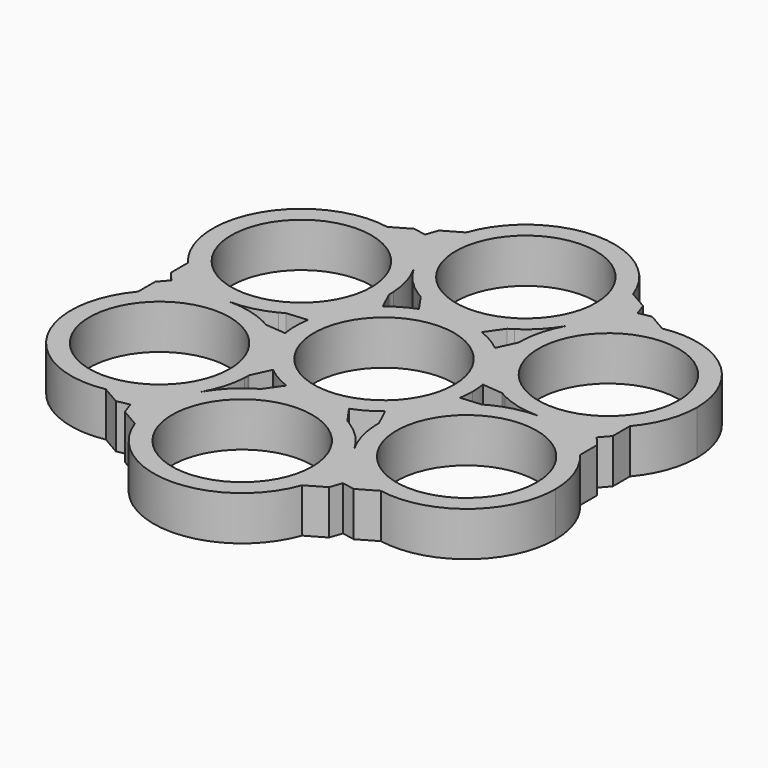
from build123d import *

# Parameters (mm, degrees)
F0_R     = 11.049
F1_DEPTH = 6.985


# Not quite as in the source:
# - a feature names something its author has since deleted; it is built from what else it names


with BuildPart() as f1:
    # F0 (on Top) → F1 (new body)
    with BuildSketch(Plane.XY):
        with BuildLine():
            ThreePointArc((13.786655701, -2.2558866507), (13.9240884826, -1.1316624621), (13.97, 0))
            ThreePointArc((13.97, 0), (13.9240884826, 1.1316624621), (13.786655701, 2.2558866507))
            ThreePointArc((13.786655701, 2.2558866507), (13.1567408564, 4.6969213362), (12.0983748352, 6.9850000964))
            ThreePointArc((12.0983748352, 6.9850000964), (10.6460235529, 9.0456112293), (8.8469829981, 10.811650745))
            ThreePointArc((8.8469829981, 10.811650745), (6.985, 12.0983748909), (4.9396727029, 13.0675373957))
            ThreePointArc((4.9396727029, 13.0675373957), (2.5107172862, 13.7425324707), (0, 13.97))
            ThreePointArc((0, 13.97), (-2.5107172862, 13.7425324707), (-4.9396727029, 13.0675373957))
            ThreePointArc((-4.9396727029, 13.0675373957), (-6.985, 12.0983748909), (-8.8469829981, 10.811650745))
            ThreePointArc((-8.8469829981, 10.811650745), (-10.6460236342, 9.0456111335), (-12.0983749609, 6.9849998787))
            ThreePointArc((-12.0983749609, 6.9849998787), (-13.1567408986, 4.6969212179), (-13.786655701, 2.2558866507))
            ThreePointArc((-13.786655701, 2.2558866507), (-13.97, 0), (-13.786655701, -2.2558866507))
            ThreePointArc((-13.786655701, -2.2558866507), (-13.1567408656, -4.6969213103), (-12.0983748628, -6.9850000487))
            ThreePointArc((-12.0983748628, -6.9850000487), (-10.6460235707, -9.0456112083), (-8.8469829981, -10.811650745))
            ThreePointArc((-8.8469829981, -10.811650745), (-6.985, -12.0983748909), (-4.9396727029, -13.0675373957))
            ThreePointArc((-4.9396727029, -13.0675373957), (-2.5107172928, -13.7425324695), (-1.35e-08, -13.97))
            ThreePointArc((-1.35e-08, -13.97), (2.5107172795, -13.7425324719), (4.9396727029, -13.0675373957))
            ThreePointArc((4.9396727029, -13.0675373957), (6.985, -12.0983748909), (8.8469829981, -10.811650745))
            ThreePointArc((8.8469829981, -10.811650745), (10.6460235529, -9.0456112293), (12.0983748352, -6.9850000964))
            ThreePointArc((12.0983748352, -6.9850000964), (13.1567408564, -4.6969213362), (13.786655701, -2.2558866507))
        make_face()
        Circle(F0_R, mode=Mode.SUBTRACT)
        with BuildLine():
            ThreePointArc((12.0983748352, 6.9850000964), (13.1567408564, 4.6969213362), (13.786655701, 2.2558866507))
            Line((13.786655701, 2.2558866507), (17.0463049997, 1.9686650985))
            ThreePointArc((17.0463049997, 1.9686650985), (14.2508878564, 4.1597639905), (12.0983748352, 6.9850000964))
        make_face()
        with BuildLine():
            Line((17.0463049997, -1.9686650985), (13.786655701, -2.2558866507))
            ThreePointArc((13.786655701, -2.2558866507), (13.1567408564, -4.6969213362), (12.0983748352, -6.9850000964))
            ThreePointArc((12.0983748352, -6.9850000964), (14.2508878564, -4.1597639905), (17.0463049997, -1.9686650985))
        make_face()
        with BuildLine():
            ThreePointArc((8.8469829981, 10.811650745), (10.6460235529, 9.0456112293), (12.0983748352, 6.9850000964))
            ThreePointArc((12.0983748352, 6.9850000964), (10.7279051882, 10.2617490221), (10.2280664867, 13.7782006212))
            Line((10.2280664867, 13.7782006212), (8.8469829981, 10.811650745))
        make_face()
        with BuildLine():
            ThreePointArc((10.2280664867, 13.7782006212), (10.7279051882, 10.2617490221), (12.0983748352, 6.9850000964))
            ThreePointArc((12.0983748352, 6.9850000964), (14.2508878564, 4.1597639905), (17.0463049997, 1.9686650985))
            ThreePointArc((17.0463049997, 1.9686650985), (17.4348836488, 1.7455136549), (17.8304191968, 1.5349392891))
            ThreePointArc((17.8304191968, 1.5349392891), (20.9223718291, 0.3891550696), (24.1967497683, 0))
            ThreePointArc((24.1967497683, 0), (30.0531688702, 1.2868120939), (34.8306887676, 4.9101853415))
            ThreePointArc((34.8306887676, 4.9101853415), (37.3062316104, 9.1427454817), (38.1667497817, 13.97))
            ThreePointArc((38.1667497817, 13.97), (33.1362668167, 24.7052659577), (21.6676896268, 27.7091686333))
            ThreePointArc((21.6676896268, 27.7091686333), (16.1409964163, 25.3834016715), (12.0983749062, 20.9550000265))
            ThreePointArc((12.0983749062, 20.9550000265), (10.7982040971, 17.9247279977), (10.244506016, 14.67412634))
            ThreePointArc((10.244506016, 14.67412634), (10.2291009922, 14.2262953244), (10.2280664867, 13.7782006212))
        make_face()
        with Locations((24.1967497817, 13.97)):
            Circle(F0_R, mode=Mode.SUBTRACT)
        with BuildLine():
            ThreePointArc((10.2280664867, -13.7782006212), (10.7279051882, -10.2617490221), (12.0983748352, -6.9850000964))
            ThreePointArc((12.0983748352, -6.9850000964), (10.6460235529, -9.0456112293), (8.8469829981, -10.811650745))
            Line((8.8469829981, -10.811650745), (10.2280664867, -13.7782006212))
        make_face()
        with BuildLine():
            ThreePointArc((17.0463049997, -1.9686650985), (14.2508878564, -4.1597639905), (12.0983748352, -6.9850000964))
            ThreePointArc((12.0983748352, -6.9850000964), (10.7279051882, -10.2617490221), (10.2280664867, -13.7782006212))
            ThreePointArc((10.2280664867, -13.7782006212), (10.2291009922, -14.2262953244), (10.244506016, -14.67412634))
            ThreePointArc((10.244506016, -14.67412634), (10.7982040928, -17.9247279832), (12.0983748911, -20.9550000004))
            ThreePointArc((12.0983748911, -20.9550000004), (16.140996404, -25.3834016628), (21.6676896268, -27.7091686333))
            ThreePointArc((21.6676896268, -27.7091686333), (33.1362668167, -24.7052659577), (38.1667497817, -13.97))
            ThreePointArc((38.1667497817, -13.97), (37.3062316104, -9.1427454817), (34.8306887676, -4.9101853415))
            ThreePointArc((34.8306887676, -4.9101853415), (30.0531688702, -1.2868120939), (24.1967497683, 0))
            ThreePointArc((24.1967497683, 0), (20.9223718291, -0.3891550696), (17.8304191968, -1.5349392891))
            ThreePointArc((17.8304191968, -1.5349392891), (17.4348836488, -1.7455136549), (17.0463049997, -1.9686650985))
        make_face()
        with Locations((24.1967497817, -13.97)):
            Circle(F0_R, mode=Mode.SUBTRACT)
        with BuildLine():
            ThreePointArc((0, 13.97), (2.5107172862, 13.7425324707), (4.9396727029, 13.0675373957))
            Line((4.9396727029, 13.0675373957), (6.818238513, 15.7468657196))
            ThreePointArc((6.818238513, 15.7468657196), (3.5229826925, 14.4215129194), (0, 13.97))
        make_face()
        with BuildLine():
            ThreePointArc((34.8306887676, 4.9101853415), (30.0531688702, 1.2868120939), (24.1967497683, 0))
            ThreePointArc((24.1967497683, 0), (30.0531688702, -1.2868120939), (34.8306887676, -4.9101853415))
            Line((34.8306887676, -4.9101853415), (34.8306887676, -1.5349392891))
            Line((34.8306887676, -1.5349392891), (33.5076935589, 0))
            Line((33.5076935589, 0), (34.8306887676, 1.5349392891))
            Line((34.8306887676, 1.5349392891), (34.8306887676, 4.9101853415))
        make_face()
        with BuildLine():
            Line((6.818238513, -15.7468657196), (4.9396727029, -13.0675373957))
            ThreePointArc((4.9396727029, -13.0675373957), (2.5107172795, -13.7425324719), (-1.35e-08, -13.97))
            ThreePointArc((-1.35e-08, -13.97), (3.5229826859, -14.4215129177), (6.818238513, -15.7468657196))
        make_face()
        with BuildLine():
            ThreePointArc((-4.9396727029, 13.0675373957), (-2.5107172862, 13.7425324707), (0, 13.97))
            ThreePointArc((0, 13.97), (-3.5229826925, 14.4215129194), (-6.818238513, 15.7468657196))
            Line((-6.818238513, 15.7468657196), (-4.9396727029, 13.0675373957))
        make_face()
        with BuildLine():
            ThreePointArc((-6.818238513, 15.7468657196), (-3.5229826925, 14.4215129194), (0, 13.97))
            ThreePointArc((0, 13.97), (3.5229826925, 14.4215129194), (6.818238513, 15.7468657196))
            ThreePointArc((6.818238513, 15.7468657196), (7.2057826566, 15.9718089794), (7.5859131808, 16.2090656291))
            ThreePointArc((7.5859131808, 16.2090656291), (10.1241677534, 18.3138830621), (12.0983749062, 20.9550000265))
            ThreePointArc((12.0983749062, 20.9550000265), (13.4939837972, 24.3242979547), (13.97, 27.94))
            ThreePointArc((13.97, 27.94), (13.7667715532, 30.314215871), (13.1629991407, 32.6193539748))
            ThreePointArc((13.1629991407, 32.6193539748), (0, 41.91), (-13.1629991407, 32.6193539748))
            ThreePointArc((-13.1629991407, 32.6193539748), (-13.9121724704, 26.670213737), (-12.0983748684, 20.9549999611))
            ThreePointArc((-12.0983748684, 20.9549999611), (-10.1241677273, 18.3138830348), (-7.5859131808, 16.2090656291))
            ThreePointArc((-7.5859131808, 16.2090656291), (-7.2057826566, 15.9718089794), (-6.818238513, 15.7468657196))
        make_face()
        with Locations((0, 27.94)):
            Circle(F0_R, mode=Mode.SUBTRACT)
        with BuildLine():
            ThreePointArc((13.97, 27.94), (13.4939837972, 24.3242979547), (12.0983749062, 20.9550000265))
            ThreePointArc((12.0983749062, 20.9550000265), (16.1409964163, 25.3834016715), (21.6676896268, 27.7091686333))
            Line((21.6676896268, 27.7091686333), (18.7446408014, 29.3967916595))
            Line((18.7446408014, 29.3967916595), (16.7538467795, 29.0185138443))
            Line((16.7538467795, 29.0185138443), (16.0860479661, 30.9317309486))
            Line((16.0860479661, 30.9317309486), (13.1629991407, 32.6193539748))
            ThreePointArc((13.1629991407, 32.6193539748), (13.7667715532, 30.314215871), (13.97, 27.94))
        make_face()
        with BuildLine():
            ThreePointArc((-6.818238513, -15.7468657196), (-3.522982699, -14.4215129211), (-1.35e-08, -13.97))
            ThreePointArc((-1.35e-08, -13.97), (-2.5107172928, -13.7425324695), (-4.9396727029, -13.0675373957))
            Line((-4.9396727029, -13.0675373957), (-6.818238513, -15.7468657196))
        make_face()
        with BuildLine():
            ThreePointArc((6.818238513, -15.7468657196), (3.5229826859, -14.4215129177), (-1.35e-08, -13.97))
            ThreePointArc((-1.35e-08, -13.97), (-3.522982699, -14.4215129211), (-6.818238513, -15.7468657196))
            ThreePointArc((-6.818238513, -15.7468657196), (-7.2057826566, -15.9718089794), (-7.5859131808, -16.2090656291))
            ThreePointArc((-7.5859131808, -16.2090656291), (-10.1241677569, -18.3138830658), (-12.0983749113, -20.9550000353))
            ThreePointArc((-12.0983749113, -20.9550000353), (-13.9121724743, -26.6702137797), (-13.1629991407, -32.6193539748))
            ThreePointArc((-13.1629991407, -32.6193539748), (0, -41.91), (13.1629991407, -32.6193539748))
            ThreePointArc((13.1629991407, -32.6193539748), (13.7667715532, -30.314215871), (13.97, -27.94))
            ThreePointArc((13.97, -27.94), (13.4939837933, -24.3242979401), (12.0983748911, -20.9550000004))
            ThreePointArc((12.0983748911, -20.9550000004), (10.124167743, -18.3138830512), (7.5859131808, -16.2090656291))
            ThreePointArc((7.5859131808, -16.2090656291), (7.2057826566, -15.9718089794), (6.818238513, -15.7468657196))
        make_face()
        with Locations((0, -27.94)):
            Circle(F0_R, mode=Mode.SUBTRACT)
        with BuildLine():
            ThreePointArc((21.6676896268, -27.7091686333), (16.140996404, -25.3834016628), (12.0983748911, -20.9550000004))
            ThreePointArc((12.0983748911, -20.9550000004), (13.4939837933, -24.3242979401), (13.97, -27.94))
            ThreePointArc((13.97, -27.94), (13.7667715532, -30.314215871), (13.1629991407, -32.6193539748))
            Line((13.1629991407, -32.6193539748), (16.0860479661, -30.9317309486))
            Line((16.0860479661, -30.9317309486), (16.7538467795, -29.0185138443))
            Line((16.7538467795, -29.0185138443), (18.7446408014, -29.3967916595))
            Line((18.7446408014, -29.3967916595), (21.6676896268, -27.7091686333))
        make_face()
        with BuildLine():
            ThreePointArc((-12.0983749609, 6.9849998787), (-10.6460236342, 9.0456111335), (-8.8469829981, 10.811650745))
            Line((-8.8469829981, 10.811650745), (-10.2280664867, 13.7782006212))
            ThreePointArc((-10.2280664867, 13.7782006212), (-10.7279052216, 10.261748901), (-12.0983749609, 6.9849998787))
        make_face()
        with BuildLine():
            Line((-10.2280664867, -13.7782006212), (-8.8469829981, -10.811650745))
            ThreePointArc((-8.8469829981, -10.811650745), (-10.6460235707, -9.0456112083), (-12.0983748628, -6.9850000487))
            ThreePointArc((-12.0983748628, -6.9850000487), (-10.7279051955, -10.2617489956), (-10.2280664867, -13.7782006212))
        make_face()
        with BuildLine():
            ThreePointArc((-13.786655701, 2.2558866507), (-13.1567408986, 4.6969212179), (-12.0983749609, 6.9849998787))
            ThreePointArc((-12.0983749609, 6.9849998787), (-14.2508879446, 4.1597639011), (-17.0463049997, 1.9686650985))
            Line((-17.0463049997, 1.9686650985), (-13.786655701, 2.2558866507))
        make_face()
        with BuildLine():
            ThreePointArc((-17.0463049997, 1.9686650985), (-14.2508879446, 4.1597639011), (-12.0983749609, 6.9849998787))
            ThreePointArc((-12.0983749609, 6.9849998787), (-10.7279052216, 10.261748901), (-10.2280664867, 13.7782006212))
            ThreePointArc((-10.2280664867, 13.7782006212), (-10.2270789618, 13.8740980508), (-10.2267497817, 13.97))
            ThreePointArc((-10.2267497817, 13.97), (-10.2311895458, 14.3221750937), (-10.244506016, 14.67412634))
            ThreePointArc((-10.244506016, 14.67412634), (-10.7982040864, 17.9247279614), (-12.0983748684, 20.9549999611))
            ThreePointArc((-12.0983748684, 20.9549999611), (-16.1409963854, 25.3834016497), (-21.6676896268, 27.7091686333))
            ThreePointArc((-21.6676896268, 27.7091686333), (-36.2951246726, 20.955), (-34.8306887676, 4.9101853415))
            ThreePointArc((-34.8306887676, 4.9101853415), (-30.0531688763, 1.2868120967), (-24.1967497817, 0))
            ThreePointArc((-24.1967497817, 0), (-20.9223718356, 0.3891550681), (-17.8304191968, 1.5349392891))
            ThreePointArc((-17.8304191968, 1.5349392891), (-17.4348836488, 1.7455136549), (-17.0463049997, 1.9686650985))
        make_face()
        with Locations((-24.1967497817, 13.97)):
            Circle(F0_R, mode=Mode.SUBTRACT)
        with BuildLine():
            ThreePointArc((-21.6676896268, 27.7091686333), (-16.1409963854, 25.3834016497), (-12.0983748684, 20.9549999611))
            ThreePointArc((-12.0983748684, 20.9549999611), (-13.9121724704, 26.670213737), (-13.1629991407, 32.6193539748))
            Line((-13.1629991407, 32.6193539748), (-16.0860479661, 30.9317309486))
            Line((-16.0860479661, 30.9317309486), (-16.7538467795, 29.0185138443))
            Line((-16.7538467795, 29.0185138443), (-18.7446408014, 29.3967916595))
            Line((-18.7446408014, 29.3967916595), (-21.6676896268, 27.7091686333))
        make_face()
        with BuildLine():
            ThreePointArc((-17.0463049997, -1.9686650985), (-14.2508878757, -4.1597639709), (-12.0983748628, -6.9850000487))
            ThreePointArc((-12.0983748628, -6.9850000487), (-13.1567408656, -4.6969213103), (-13.786655701, -2.2558866507))
            Line((-13.786655701, -2.2558866507), (-17.0463049997, -1.9686650985))
        make_face()
        with BuildLine():
            ThreePointArc((-10.2280664867, -13.7782006212), (-10.7279051955, -10.2617489956), (-12.0983748628, -6.9850000487))
            ThreePointArc((-12.0983748628, -6.9850000487), (-14.2508878757, -4.1597639709), (-17.0463049997, -1.9686650985))
            ThreePointArc((-17.0463049997, -1.9686650985), (-17.4348836488, -1.7455136549), (-17.8304191968, -1.5349392891))
            ThreePointArc((-17.8304191968, -1.5349392891), (-20.9223718356, -0.3891550681), (-24.1967497817, 0))
            ThreePointArc((-24.1967497817, 0), (-30.0531688763, -1.2868120967), (-34.8306887676, -4.9101853415))
            ThreePointArc((-34.8306887676, -4.9101853415), (-36.2951246726, -20.955), (-21.6676896268, -27.7091686333))
            ThreePointArc((-21.6676896268, -27.7091686333), (-16.1409964205, -25.3834016745), (-12.0983749113, -20.9550000353))
            ThreePointArc((-12.0983749113, -20.9550000353), (-10.7982040985, -17.9247280026), (-10.244506016, -14.67412634))
            ThreePointArc((-10.244506016, -14.67412634), (-10.2311895458, -14.3221750937), (-10.2267497817, -13.97))
            ThreePointArc((-10.2267497817, -13.97), (-10.2270789618, -13.8740980508), (-10.2280664867, -13.7782006212))
        make_face()
        with Locations((-24.1967497817, -13.97)):
            Circle(F0_R, mode=Mode.SUBTRACT)
        with BuildLine():
            ThreePointArc((-13.1629991407, -32.6193539748), (-13.9121724743, -26.6702137797), (-12.0983749113, -20.9550000353))
            ThreePointArc((-12.0983749113, -20.9550000353), (-16.1409964205, -25.3834016745), (-21.6676896268, -27.7091686333))
            Line((-21.6676896268, -27.7091686333), (-18.7446408014, -29.3967916595))
            Line((-18.7446408014, -29.3967916595), (-16.7538467795, -29.0185138443))
            Line((-16.7538467795, -29.0185138443), (-16.0860479661, -30.9317309486))
            Line((-16.0860479661, -30.9317309486), (-13.1629991407, -32.6193539748))
        make_face()
        with BuildLine():
            ThreePointArc((-24.1967497817, 0), (-30.0531688763, 1.2868120967), (-34.8306887676, 4.9101853415))
            Line((-34.8306887676, 4.9101853415), (-34.8306887676, 1.5349392891))
            Line((-34.8306887676, 1.5349392891), (-33.5076935589, 0))
            Line((-33.5076935589, 0), (-34.8306887676, -1.5349392891))
            Line((-34.8306887676, -1.5349392891), (-34.8306887676, -4.9101853415))
            ThreePointArc((-34.8306887676, -4.9101853415), (-30.0531688763, -1.2868120967), (-24.1967497817, 0))
        make_face()
    extrude(amount=F1_DEPTH)


solid = f1.part
